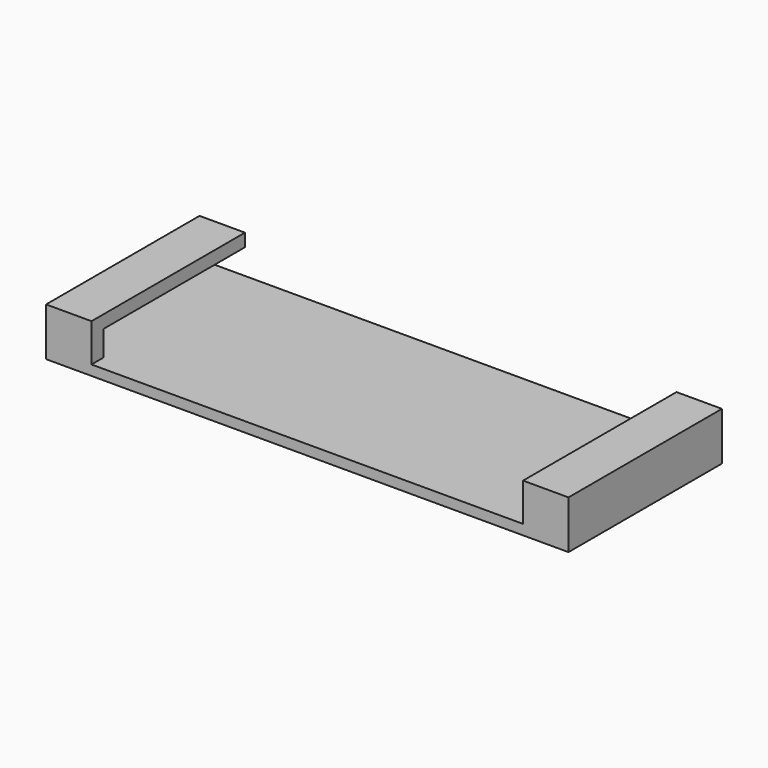
from build123d import *

# Parameters (mm, degrees)
F0_W     = 98.5
F0_H     = 38
F1_DEPTH = 2
F3_DEPTH = 35
F4_W     = 9
F4_H     = 9.55
F5_DEPTH = 3
F6_R     = 1.5
F7_DEPTH = 1.5
F8_R     = 0.74999


# Not quite as in the source:
# - a fillet or chamfer is up to 0.001 mm smaller than in the source, because OpenCascade refuses the exact size


with BuildPart() as f1:
    # F0 (on Top) → F1 (new body)
    with BuildSketch(Plane.XY):
        with Locations((49.25, 19)):
            Rectangle(F0_W, F0_H)
    extrude(amount=F1_DEPTH)

    # F2 (on face) → F3 (join)
    with BuildSketch(Plane(origin=(0, 38, 0), x_dir=(-1, 0, 0), z_dir=(0, 1, 0))):
        Polygon((-101, 0), (-98.5, 0), (-98.5, 7), (-92, 7), (-92, 9.55), (-101, 9.55), align=None)
        Polygon((0, 7), (0, 0), (2.5, 0), (2.5, 9.55), (-6.5, 9.55), (-6.5, 7), align=None)
    extrude(amount=-F3_DEPTH)

    # F4 (on face) → F5 (join)
    with BuildSketch(Plane.XZ.offset(-3)):
        with Locations((2, 4.775)):
            Rectangle(F4_W, F4_H)
        with Locations((96.5, 4.775)):
            Rectangle(F4_W, F4_H)
    extrude(amount=F5_DEPTH)

    # F6 (on face) → F7 (join)
    with BuildSketch(Plane.YZ):
        with Locations((6.5, 4.25)):
            Circle(F6_R)
    extrude(amount=F7_DEPTH)

    # F8 (radius 0.75 in the source; OpenCascade refuses exactly that, so slightly less here)
    f8_edges = [f1.edges().sort_by_distance(p)[0] for p in [
        (1.5, 5, 4.25),
        (0, 5, 4.25),
    ]]
    fillet(f8_edges, radius=F8_R)


solid = f1.part
